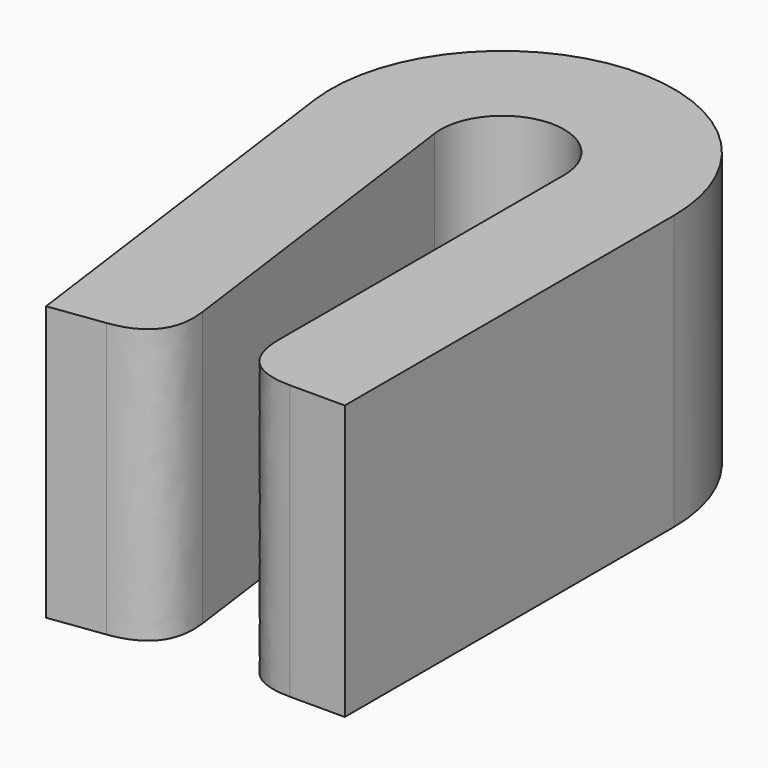
from build123d import *

# Parameters (mm, degrees)
F1_DEPTH    = 10
F2_T1_DEPTH = 20


# Not quite as in the source:
# - a fillet or chamfer that OpenCascade refuses, or shapes differently, is made with other operations: its cross-section is extruded or revolved along the edge and cut away or added


with BuildPart() as f1:
    # F0 (on Top) → F1 (new body)
    with BuildSketch(Plane.XY):
        with BuildLine():
            ThreePointArc((-2.2298651391, -0.300335581), (-0.1505048785, 2.2449606414), (2.25, 0))
            Line((2.25, 0), (2.25, -15))
            Line((2.25, -15), (6.25, -15))
            Line((6.25, -15), (6.25, 0))
            ThreePointArc((6.25, 0), (-0.418069107, 6.2360017817), (-6.194069831, -0.8342655028))
            Line((-6.194069831, -0.8342655028), (-4.2142046918, -15.5339299218))
            Line((-4.2142046918, -15.5339299218), (-0.25, -15))
            Line((-0.25, -15), (-2.2298651391, -0.300335581))
        make_face()
    extrude(amount=F1_DEPTH)

    # F2: fillet of radius 2 on 2 edges, made by hand

    # F2_s2 → F2_t1 (cut)
    with BuildSketch(Plane.XY.offset(-5)):
        with BuildLine():
            add(Edge.make_bspline(
                [(-2.2321023459, -15.2669649609), (-0.25, -15), (-0.5169649609, -13.0178976541)],
                knots=[0, 0, 0, 1, 1, 1], degree=2, weights=[1, 1, 1]))
            Line((-0.5169649609, -13.0178976541), (-0.25, -15))
            Line((-0.25, -15), (-2.2321023459, -15.2669649609))
        make_face()
        with BuildLine():
            add(Edge.make_bspline(
                [(2.25, -13), (2.25, -15), (4.25, -15)],
                knots=[0, 0, 0, 1, 1, 1], degree=2, weights=[1, 1, 1]))
            Line((4.25, -15), (2.25, -15))
            Line((2.25, -15), (2.25, -13))
        make_face()
    extrude(amount=F2_T1_DEPTH, mode=Mode.SUBTRACT)


solid = f1.part
